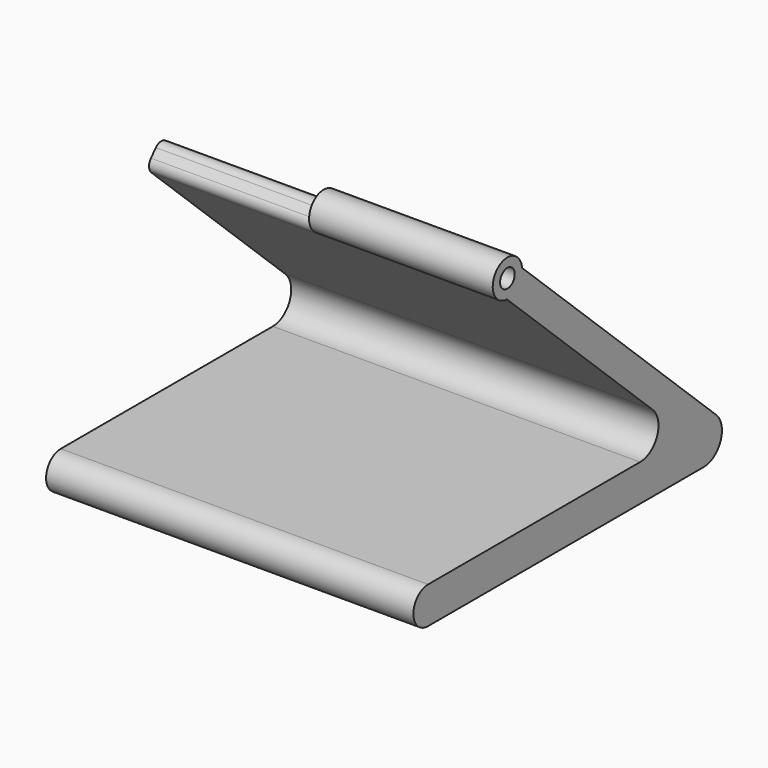
from build123d import *

# Parameters (mm, degrees)
F1_DEPTH    = 40
F4_DEPTH    = 40
F7_D        = 4
F8_T1_DEPTH = 45.0963937419
F8_T3_DEPTH = 44.9054294597


# Not quite as in the source:
# - a fillet or chamfer that OpenCascade refuses, or shapes differently, is made with other operations: its cross-section is extruded or revolved along the edge and cut away or added


with BuildPart() as f1:
    # F0 (on Right) → F1 (new body)
    with BuildSketch(Plane.YZ):
        with BuildLine():
            ThreePointArc((-63.4816033854, -7.334386461), (-67.4816033854, -11.334386461), (-63.4816033854, -15.334386461))
            Line((-63.4816033854, -15.334386461), (11.5183966146, -15.334386461))
            ThreePointArc((11.5183966146, -15.334386461), (16.1842937846, -12.1314406057), (14.8723445539, -6.6261479006))
            Line((14.8723445539, -6.6261479006), (-36.2252883959, 41.3947367846))
            Line((-36.2252883959, 41.3947367846), (-40.2507597139, 36.9440392082))
            Line((-40.2507597139, 36.9440392082), (-2.4015535455, 1.3738520994))
            ThreePointArc((-2.4015535455, 1.3738520994), (-1.0896043148, -4.1314406057), (-5.7555014847, -7.334386461))
            Line((-5.7555014847, -7.334386461), (-63.4816033854, -7.334386461))
        make_face()
    extrude(amount=F1_DEPTH)

    # F3 (on offset) → F4 (join)
    with BuildSketch(Plane.YZ.offset(40)):
        with BuildLine():
            Line((14.8723445539, -6.6261479006), (-36.2252883959, 41.3947367846))
            Line((-36.2252883959, 41.3947367846), (-40.2507597139, 36.9440392082))
            Line((-40.2507597139, 36.9440392082), (-2.4015535455, 1.3738520994))
            ThreePointArc((-2.4015535455, 1.3738520994), (-1.0896043148, -4.1314406057), (-5.7555014847, -7.334386461))
            Line((-5.7555014847, -7.334386461), (-63.4816033854, -7.334386461))
            ThreePointArc((-63.4816033854, -7.334386461), (-67.4816033854, -11.334386461), (-63.4816033854, -15.334386461))
            Line((-63.4816033854, -15.334386461), (11.5183966146, -15.334386461))
            ThreePointArc((11.5183966146, -15.334386461), (16.1842937846, -12.1314406057), (14.8723445539, -6.6261479006))
        make_face()
        with BuildLine():
            Line((-40.2507597139, 36.9440392082), (-36.2252883959, 41.3947367846))
            Line((-36.2252883959, 41.3947367846), (-37.8997588755, 42.9683821605))
            ThreePointArc((-37.8997588755, 42.9683821605), (-37.8866027682, 42.7814716227), (-37.8822141892, 42.5941500472))
            ThreePointArc((-37.8822141892, 42.5941500472), (-39.0988744687, 39.7213430575), (-42.0087241892, 38.5961511452))
            Line((-42.0087241892, 38.5961511452), (-40.2507597139, 36.9440392082))
        make_face()
        with BuildLine():
            ThreePointArc((-37.8822141892, 42.5941500472), (-37.8866027682, 42.7814716227), (-37.8997588755, 42.9683821605))
            ThreePointArc((-37.8997588755, 42.9683821605), (-44.7970348661, 45.3334602563), (-42.0087241892, 38.5961511452))
            ThreePointArc((-42.0087241892, 38.5961511452), (-39.0988744687, 39.7213430575), (-37.8822141892, 42.5941500472))
        make_face()
    extrude(amount=F4_DEPTH)

    # F7 (through all)
    with Locations(Plane.YZ.offset(120)):
        with Locations((-41.8822141892, 42.5941500472)):
            Hole(F7_D / 2)

    # F8: fillet of radius 2 on 2 edges, made by hand

    # F8_s2 → F8_t1 (cut)
    with BuildSketch(Plane.YZ.offset(-5.0963937419)):
        with BuildLine():
            ThreePointArc((-37.592731539, 39.8828452812), (-36.190570233, 40.5396197416), (-34.7397810103, 39.9986764439))
            Line((-34.7397810103, 39.9986764439), (-36.2252883959, 41.3947367846))
            Line((-36.2252883959, 41.3947367846), (-37.592731539, 39.8828452812))
        make_face()
    extrude(amount=F8_T1_DEPTH, mode=Mode.SUBTRACT)

    # F8_s4 → F8_t3 (cut)
    with BuildSketch(Plane.YZ.offset(-4.9054294597)):
        with BuildLine():
            ThreePointArc((-38.9345553117, 38.3992794224), (-39.4496135236, 36.9765661286), (-38.8209149921, 35.6002899083))
            Line((-38.8209149921, 35.6002899083), (-40.2507597139, 36.9440392082))
            Line((-40.2507597139, 36.9440392082), (-38.9345553117, 38.3992794224))
        make_face()
    extrude(amount=F8_T3_DEPTH, mode=Mode.SUBTRACT)


solid = f1.part
